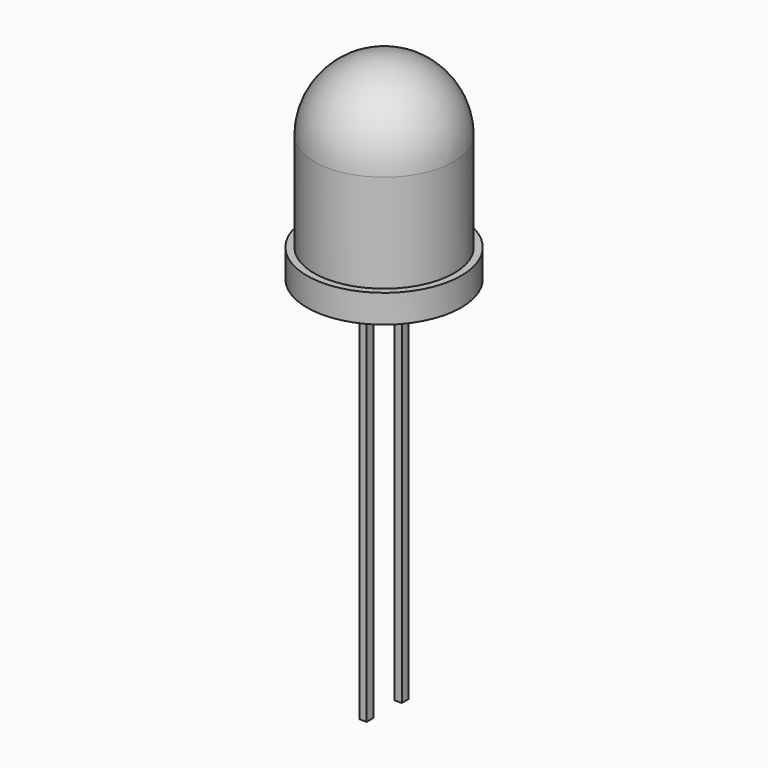
from build123d import *

# Parameters (mm, degrees)
F0_R     = 5
F1_DEPTH = 7
F4_R     = 5.5
F4_R_2   = 5
F5_DEPTH = 2
F7_DEPTH = 28
F8_DEPTH = 26


with BuildPart() as f1:
    # F0 (on Top) → F1 (new body)
    with BuildSketch(Plane.XY):
        Circle(F0_R)
    extrude(amount=F1_DEPTH)

    # F2 (on Front) → F3 (revolve)
    with BuildSketch(Plane.XZ):
        with BuildLine():
            Line((0, 12), (0, 7))
            Line((0, 7), (5, 7))
            ThreePointArc((5, 7), (3.5355339059, 10.5355339059), (0, 12))
        make_face()
    revolve(axis=Axis((0, 0, 10.5024230517), (0, 0, -1)))

    # F4 (on face) → F5 (join)
    with BuildSketch(Plane(origin=(0, 0, 0), x_dir=(1, 0, 0), z_dir=(0, 0, -1))):
        Circle(F4_R)
        Circle(F4_R_2, mode=Mode.SUBTRACT)
        Circle(F4_R_2)
    extrude(amount=F5_DEPTH)

    # F6 (on face) → F7 (join)
    with BuildSketch(Plane(origin=(0, 0, -2), x_dir=(1, 0, 0), z_dir=(0, 0, -1))):
        Polygon((-1, -0.3), (-1, 0), (-1, 0.3), (-1.5, 0.3), (-1.5, -0.3), align=None)
    extrude(amount=F7_DEPTH)

    # F6 (on face) → F8 (join)
    with BuildSketch(Plane(origin=(0, 0, -2), x_dir=(1, 0, 0), z_dir=(0, 0, -1))):
        Polygon((1, 0.3), (1, 0), (1, -0.3), (1.5, -0.3), (1.5, 0.3), align=None)
    extrude(amount=F8_DEPTH)


solid = f1.part
